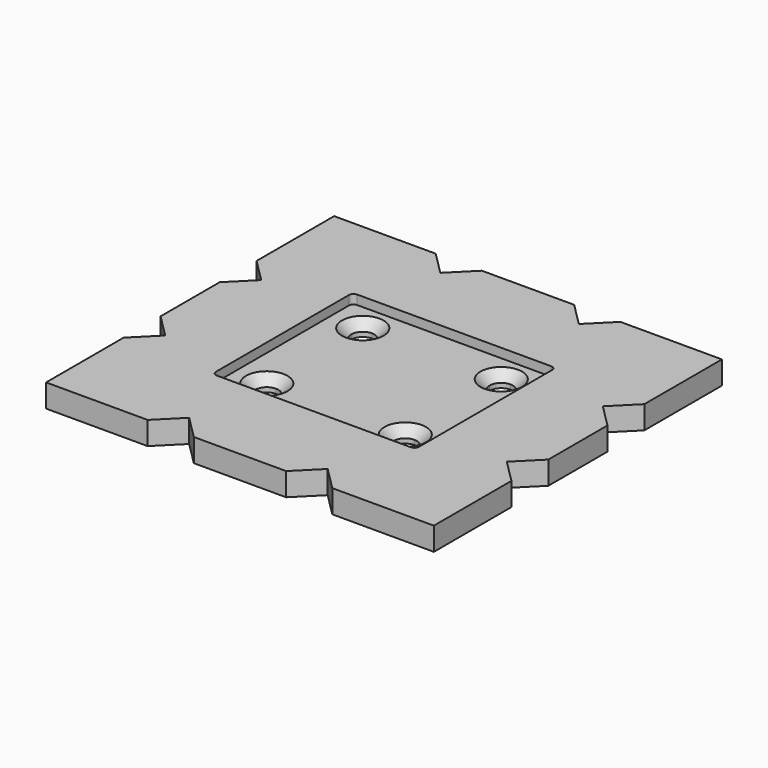
from build123d import *

# Parameters (mm, degrees)
F1_DEPTH = 3
F4_DEPTH = 5
F5_R     = 1


# Not quite as in the source:
# - a fillet or chamfer that OpenCascade refuses, or shapes differently, is made with other operations: its cross-section is extruded or revolved along the edge and cut away or added
# - a feature of the source that left no trace in its solid (it failed there, or was rolled back) is left out


with BuildPart() as f1:
    # F0 (on Top) → F1 (new body)
    with BuildSketch(Plane.XY):
        Polygon((-22, -13), (-22, 13), (-37, 13), (-42, 8), (-42, -8), (-37, -13), align=None)
        with BuildLine():
            Line((-15, -10.5), (-15, 10.5))
            ThreePointArc((-15, 10.5), (-16.767766953, 11.232233047), (-17.5, 13))
            Line((-17.5, 13), (-22, 13))
            Line((-22, 13), (-22, -13))
            Line((-22, -13), (-17.5, -13))
            ThreePointArc((-17.5, -13), (-16.767766953, -11.232233047), (-15, -10.5))
        make_face()
        Polygon((37, 13), (22, 13), (22, -13), (37, -13), (42, -8), (42, 8), align=None)
        with BuildLine():
            Line((15, 19), (15, 15.5))
            ThreePointArc((15, 15.5), (16.767766953, 14.767766953), (17.5, 13))
            Line((17.5, 13), (22, 13))
            Line((22, 13), (22, 19))
            Line((22, 19), (15, 19))
        make_face()
        with BuildLine():
            Line((22, -13), (17.5, -13))
            ThreePointArc((17.5, -13), (16.767766953, -14.767766953), (15, -15.5))
            Line((15, -15.5), (15, -19))
            Line((15, -19), (22, -19))
            Line((22, -19), (22, -13))
        make_face()
        with BuildLine():
            Line((12.5, 13), (-12.5, 13))
            ThreePointArc((-12.5, 13), (-13.232233047, 11.232233047), (-15, 10.5))
            Line((-15, 10.5), (-15, -10.5))
            ThreePointArc((-15, -10.5), (-13.232233047, -11.232233047), (-12.5, -13))
            Line((-12.5, -13), (12.5, -13))
            ThreePointArc((12.5, -13), (13.232233047, -11.232233047), (15, -10.5))
            Line((15, -10.5), (15, 10.5))
            ThreePointArc((15, 10.5), (13.232233047, 11.232233047), (12.5, 13))
        make_face()
        with BuildLine():
            ThreePointArc((-15, -15.5), (-16.767766953, -14.767766953), (-17.5, -13))
            Line((-17.5, -13), (-22, -13))
            Line((-22, -13), (-22, -19))
            Line((-22, -19), (-15, -19))
            Line((-15, -19), (-15, -15.5))
        make_face()
        Polygon((-15, 34), (-15, 19), (15, 19), (15, 34), (10, 39), (-10, 39), align=None)
        Polygon((15, -19), (-15, -19), (-15, -34), (-10, -39), (10, -39), (15, -34), align=None)
        Polygon((-22, -19), (-22, -13), (-37, -13), (-42, -18), (-42, -39), (-20, -39), (-15, -34), (-15, -19), align=None)
        Polygon((-22, 19), (-15, 19), (-15, 34), (-20, 39), (-42, 39), (-42, 18), (-37, 13), (-22, 13), align=None)
        Polygon((15, 34), (15, 19), (22, 19), (22, 13), (37, 13), (42, 18), (42, 39), (20, 39), align=None)
        Polygon((37, -13), (22, -13), (22, -19), (15, -19), (15, -34), (20, -39), (42, -39), (42, -18), align=None)
        with BuildLine():
            ThreePointArc((-17.5, 13), (-16.767766953, 14.767766953), (-15, 15.5))
            Line((-15, 15.5), (-15, 19))
            Line((-15, 19), (-22, 19))
            Line((-22, 19), (-22, 13))
            Line((-22, 13), (-17.5, 13))
        make_face()
        with BuildLine():
            Line((12.5, -13), (-12.5, -13))
            ThreePointArc((-12.5, -13), (-13.232233047, -14.767766953), (-15, -15.5))
            Line((-15, -15.5), (-15, -19))
            Line((-15, -19), (15, -19))
            Line((15, -19), (15, -15.5))
            ThreePointArc((15, -15.5), (13.232233047, -14.767766953), (12.5, -13))
        make_face()
        with BuildLine():
            ThreePointArc((-15, 15.5), (-13.232233047, 14.767766953), (-12.5, 13))
            Line((-12.5, 13), (12.5, 13))
            ThreePointArc((12.5, 13), (13.232233047, 14.767766953), (15, 15.5))
            Line((15, 15.5), (15, 19))
            Line((15, 19), (-15, 19))
            Line((-15, 19), (-15, 15.5))
        make_face()
        with BuildLine():
            ThreePointArc((17.5, 13), (16.767766953, 11.232233047), (15, 10.5))
            Line((15, 10.5), (15, -10.5))
            ThreePointArc((15, -10.5), (16.767766953, -11.232233047), (17.5, -13))
            Line((17.5, -13), (22, -13))
            Line((22, -13), (22, 13))
            Line((22, 13), (17.5, 13))
        make_face()
    extrude(amount=F1_DEPTH)

    # F2: chamfer of 2 on 4 edges, made by hand

    # F2_s1 → F2_t2 (revolve, cut)
    with BuildSketch(Plane.XZ.offset(13)):
        Polygon((-12.5, 1), (-10.5, 3), (-12.5, 3), align=None)
    revolve(axis=Axis((-15, -13, 3), (0, 0, -1)), mode=Mode.SUBTRACT)

    # F2_s3 → F2_t4 (revolve, cut)
    with BuildSketch(Plane.YZ.offset(-15)):
        Polygon((15.5, 1), (17.5, 3), (15.5, 3), align=None)
    revolve(axis=Axis((-15, 13, 3), (0, 0, -1)), mode=Mode.SUBTRACT)

    # F2_s5 → F2_t6 (revolve, cut)
    with BuildSketch(Plane.XZ.offset(-13)):
        Polygon((17.5, 1), (19.5, 3), (17.5, 3), align=None)
    revolve(axis=Axis((15, 13, 3), (0, 0, -1)), mode=Mode.SUBTRACT)

    # F2_s7 → F2_t8 (revolve, cut)
    with BuildSketch(Plane.YZ.offset(15)):
        Polygon((-10.5, 1), (-8.5, 3), (-10.5, 3), align=None)
    revolve(axis=Axis((15, -13, 3), (0, 0, -1)), mode=Mode.SUBTRACT)

    # F0 (on Top) → F4 (join)
    with BuildSketch(Plane.XY):
        Polygon((-22, 19), (-15, 19), (-15, 34), (-20, 39), (-42, 39), (-42, 18), (-37, 13), (-22, 13), align=None)
        Polygon((-22, -13), (-22, 13), (-37, 13), (-42, 8), (-42, -8), (-37, -13), align=None)
        Polygon((-22, -19), (-22, -13), (-37, -13), (-42, -18), (-42, -39), (-20, -39), (-15, -34), (-15, -19), align=None)
        Polygon((15, -19), (-15, -19), (-15, -34), (-10, -39), (10, -39), (15, -34), align=None)
        Polygon((37, -13), (22, -13), (22, -19), (15, -19), (15, -34), (20, -39), (42, -39), (42, -18), align=None)
        Polygon((37, 13), (22, 13), (22, -13), (37, -13), (42, -8), (42, 8), align=None)
        Polygon((15, 34), (15, 19), (22, 19), (22, 13), (37, 13), (42, 18), (42, 39), (20, 39), align=None)
        Polygon((-15, 34), (-15, 19), (15, 19), (15, 34), (10, 39), (-10, 39), align=None)
    extrude(amount=F4_DEPTH)

    # F5
    f5_edges = [f1.edges().sort_by_distance(p)[0] for p in [
        (-22, 19, 4),
        (-22, -19, 4),
        (22, 19, 4),
        (22, -19, 4),
    ]]
    fillet(f5_edges, radius=F5_R)


solid = f1.part
